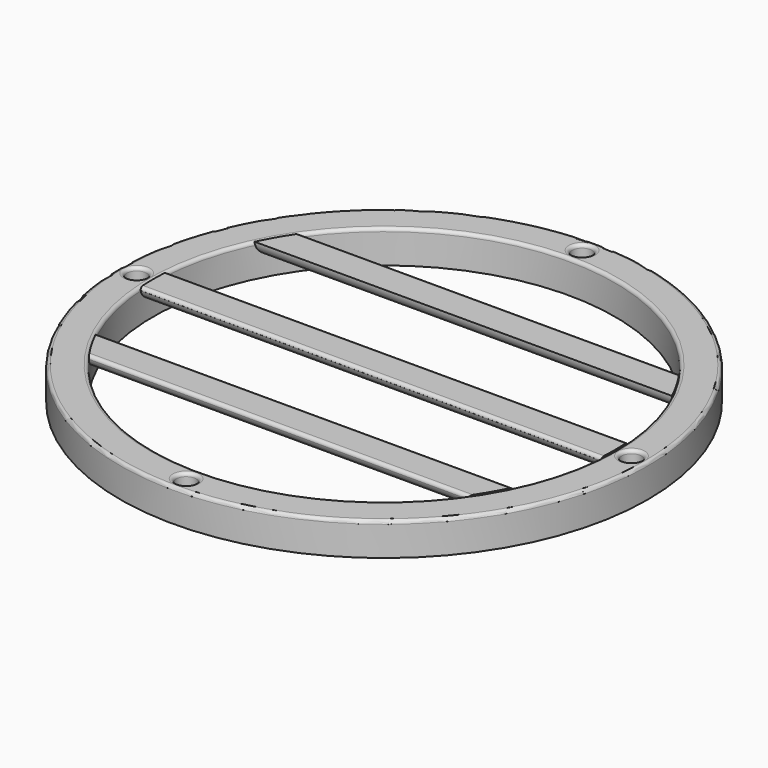
from build123d import *

# Parameters (mm, degrees)
F0_R           = 40
F0_R_2         = 35
F1_DEPTH       = 5
F3_DEPTH       = 2
F5_D           = 2
F5_CBORE_D     = 3
F5_CBORE_DEPTH = 2
F6_R           = 0.49999
F6_2_R         = 0.49999
F6_3_R         = 0.49999
F6_4_R         = 0.49999
F7_T1_DEPTH    = 73.2455532034
F7_T3_DEPTH    = 67.1280977407
F7_2_T1_DEPTH  = 79.5036714942
F7_3_T1_DEPTH  = 67.1280977407
F7_3_T3_DEPTH  = 72.9280244787


# Not quite as in the source:
# - a fillet or chamfer that OpenCascade refuses, or shapes differently, is made with other operations: its cross-section is extruded or revolved along the edge and cut away or added
# - a fillet or chamfer is up to 0.001 mm smaller than in the source, because OpenCascade refuses the exact size


with BuildPart() as f1:
    # F0 (on Top) → F1 (new body)
    with BuildSketch(Plane.XY):
        Circle(F0_R)
        Circle(F0_R_2, mode=Mode.SUBTRACT)
    extrude(amount=F1_DEPTH)

    # F5 (through all)
    with Locations(Plane.XY.offset(5)):
        with Locations((0, 37.5), (37.5, 0), (-37.5, 0), (0, -37.5)):
            CounterBoreHole(F5_D / 2, F5_CBORE_D / 2, F5_CBORE_DEPTH)

    # F6 (radius 0.5 in the source; OpenCascade refuses exactly that, so slightly less here)
    f6_edges = [f1.edges().sort_by_distance(p)[0] for p in [
        (-40, 0, 5),
        (-35, 0, 5),
        (-1.5, -37.5, 5),
        (-39, 0, 5),
        (36, 0, 5),
        (-1.5, 37.5, 5),
    ]]
    fillet(f6_edges, radius=F6_R)


with BuildPart() as f3:
    # F2 (on face) → F3 (new body)
    with BuildSketch(Plane.XY.offset(5)):
        with BuildLine():
            Line((28.7228132327, 20), (-28.7228132327, 20))
            ThreePointArc((-28.7228132327, 20), (-30.2761878894, 17.5599671664), (-31.6227766017, 15))
            Line((-31.6227766017, 15), (31.6227766017, 15))
            ThreePointArc((31.6227766017, 15), (30.2761878894, 17.5599671664), (28.7228132327, 20))
        make_face()
    extrude(amount=-F3_DEPTH)

    # F6#2 (radius 0.5 in the source; OpenCascade refuses exactly that, so slightly less here)
    f6_2_edges = [f3.edges().sort_by_distance(p)[0] for p in [
        (0, 20, 5),
    ]]
    fillet(f6_2_edges, radius=F6_2_R)

    # F7: fillet of radius 2 on 2 edges, made by hand

    # F7_s2 → F7_t1 (cut)
    with BuildSketch(Plane.YZ.offset(-36.6227766017)):
        with BuildLine():
            ThreePointArc((17, 3), (15.5857864376, 3.5857864376), (15, 5))
            Line((15, 5), (15, 3))
            Line((15, 3), (17, 3))
        make_face()
    extrude(amount=F7_T1_DEPTH, mode=Mode.SUBTRACT)

    # F7_s4 → F7_t3 (cut)
    with BuildSketch(Plane.YZ.offset(-33.5640488704)):
        with BuildLine():
            ThreePointArc((20, 4.50001), (19.2882546988, 3.4188643322), (18.0635057449, 3))
            Line((18.0635057449, 3), (20, 3))
            Line((20, 3), (20, 4.50001))
        make_face()
    extrude(amount=F7_T3_DEPTH, mode=Mode.SUBTRACT)


with BuildPart() as f3b:
    # F2 (on face) → F3, piece 2 (new body)
    with BuildSketch(Plane.XY.offset(5)):
        with BuildLine():
            Line((34.9106001094, 2.5), (-34.9106001094, 2.5))
            ThreePointArc((-34.9106001094, 2.5), (-35, 0), (-34.9106001094, -2.5))
            Line((-34.9106001094, -2.5), (34.9106001094, -2.5))
            ThreePointArc((34.9106001094, -2.5), (34.9776428868, -1.2507989787), (35, 0))
            ThreePointArc((35, 0), (34.9776428868, 1.2507989787), (34.9106001094, 2.5))
        make_face()
    extrude(amount=-F3_DEPTH)

    # F6#3 (radius 0.5 in the source; OpenCascade refuses exactly that, so slightly less here)
    f6_3_edges = [f3b.edges().sort_by_distance(p)[0] for p in [
        (0, -2.5, 5),
        (0, 2.5, 5),
    ]]
    fillet(f6_3_edges, radius=F6_3_R)

    # F7#2: fillet of radius 2 on 2 edges, made by hand

    # F7_2_s2 → F7_2_t1 (cut)
    with BuildSketch(Plane.YZ.offset(-39.7518357471)):
        with BuildLine():
            ThreePointArc((-2.5, 4.50001), (-1.7882546988, 3.4188643322), (-0.5635057449, 3))
            Line((-0.5635057449, 3), (-2.5, 3))
            Line((-2.5, 3), (-2.5, 4.50001))
        make_face()
        with BuildLine():
            ThreePointArc((0.5635057449, 3), (1.7882546988, 3.4188643322), (2.5, 4.50001))
            Line((2.5, 4.50001), (2.5, 3))
            Line((2.5, 3), (0.5635057449, 3))
        make_face()
    extrude(amount=F7_2_T1_DEPTH, mode=Mode.SUBTRACT)


with BuildPart() as f3c:
    # F2 (on face) → F3, piece 3 (new body)
    with BuildSketch(Plane.XY.offset(5)):
        with BuildLine():
            Line((31.6227766017, -15), (-31.6227766017, -15))
            ThreePointArc((-31.6227766017, -15), (-30.2761878894, -17.5599671664), (-28.7228132327, -20))
            Line((-28.7228132327, -20), (28.7228132327, -20))
            ThreePointArc((28.7228132327, -20), (30.2761878894, -17.5599671664), (31.6227766017, -15))
        make_face()
    extrude(amount=-F3_DEPTH)

    # F6#4 (radius 0.5 in the source; OpenCascade refuses exactly that, so slightly less here)
    f6_4_edges = [f3c.edges().sort_by_distance(p)[0] for p in [
        (0, -20, 5),
        (0, -15, 5),
    ]]
    fillet(f6_4_edges, radius=F6_4_R)

    # F7#3: fillet of radius 2 on 2 edges, made by hand

    # F7_3_s2 → F7_3_t1 (cut)
    with BuildSketch(Plane.YZ.offset(-33.5640488704)):
        with BuildLine():
            ThreePointArc((-20, 4.50001), (-19.2882546988, 3.4188643322), (-18.0635057449, 3))
            Line((-18.0635057449, 3), (-20, 3))
            Line((-20, 3), (-20, 4.50001))
        make_face()
    extrude(amount=F7_3_T1_DEPTH, mode=Mode.SUBTRACT)

    # F7_3_s4 → F7_3_t3 (cut)
    with BuildSketch(Plane.YZ.offset(-36.4640122393)):
        with BuildLine():
            ThreePointArc((-16.9364942551, 3), (-15.7117453012, 3.4188643322), (-15, 4.50001))
            Line((-15, 4.50001), (-15, 3))
            Line((-15, 3), (-16.9364942551, 3))
        make_face()
    extrude(amount=F7_3_T3_DEPTH, mode=Mode.SUBTRACT)


solid = Compound([f1.part, f3.part, f3b.part, f3c.part])
